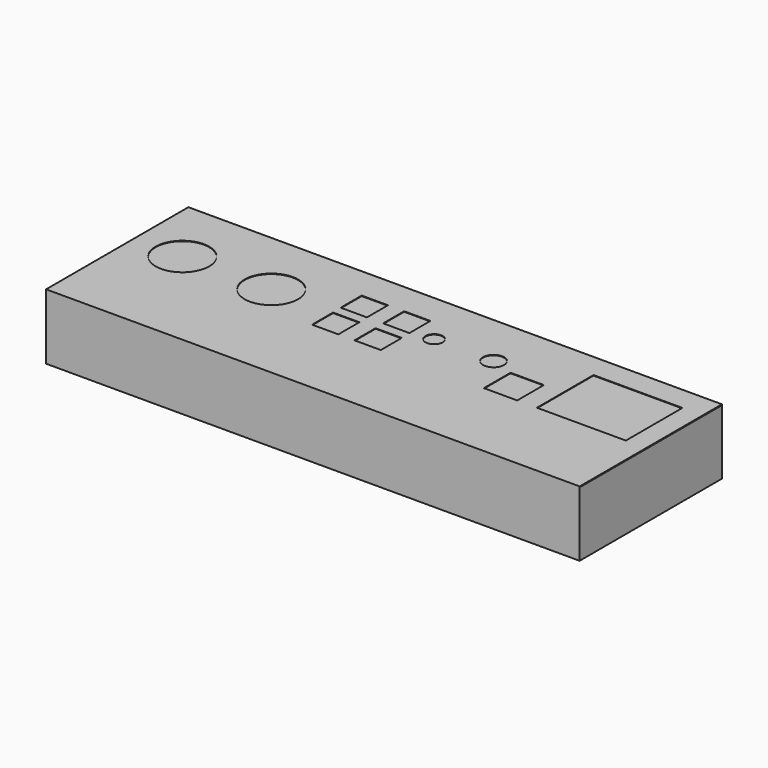
from build123d import *

# Parameters (mm, degrees)
F1_DEPTH = 209.55
F2_W     = 20.6375
F2_H     = 20.6375
F2_W_2   = 20.6374746
F2_W_3   = 69.85
F2_H_2   = 55.5625
F2_W_4   = 26.19375
F2_H_3   = 26.19375
F3_DEPTH = 0.4064


# Not quite as in the source:
# - the dataset's text gives a spline's control points without its knots; the knots are read off the source's solid


with BuildPart() as f1:
    # F0 (on Right) → F1 (new body, symmetric)
    with BuildSketch(Plane.YZ):
        Polygon((-139.7, 0), (0, 0), (0, 50.8), (-139.2936, 50.8), (-139.2936, 51.054), (0, 51.054), (0, 51.4604), (-139.7, 51.4604), align=None)
    extrude(amount=F1_DEPTH, both=True)

    # F2 (on face) → F3 (cut, through all)
    with BuildSketch(Plane.XY.offset(51.4604)):
        with Locations((-42.494652462, -64.131877524)):
            Rectangle(F2_W, F2_H)
        with Locations((-42.891171862, -35.556877524)):
            Rectangle(F2_W, F2_H)
        with Locations((-9.157152462, -64.131877524)):
            Rectangle(F2_W, F2_H)
        with Locations((-9.553684562, -35.556877524)):
            Rectangle(F2_W_2, F2_H)
        with Locations((158.720972538, -46.669377524)):
            Rectangle(F2_W_3, F2_H_2)
        with Locations((95.220972538, -61.353752524)):
            Rectangle(F2_W_4, F2_H_3)
        with BuildLine():
            add(Edge.make_bspline(
                [(22.455052538, -37.929872524), (21.206185338, -36.680675124), (19.450918338, -35.953752524), (17.684246738, -35.953752524)],
                knots=[7, 7, 7, 7, 8, 8, 8, 8], degree=3))
            add(Edge.make_bspline(
                [(17.684246738, -35.953752524), (15.918311738, -35.953752524), (14.163044738, -36.680675124), (12.913847338, -37.929872524)],
                knots=[0, 0, 0, 0, 1, 1, 1, 1], degree=3))
            add(Edge.make_bspline(
                [(12.913847338, -37.929872524), (11.664980138, -39.178384124), (10.937371738, -40.933981324), (10.937371738, -42.700627524), (10.937371738, -44.466587924), (11.664980138, -46.222235924), (12.913847338, -47.471407924)],
                knots=[1, 1, 1, 1, 2, 2, 2, 3, 3, 3, 3], degree=3))
            add(Edge.make_bspline(
                [(12.913847338, -47.471407924), (14.163044738, -48.719894124), (15.918311738, -49.447502524), (17.684246738, -49.447502524), (19.450918338, -49.447502524), (21.206185338, -48.719894124), (22.455052538, -47.471407924)],
                knots=[3, 3, 3, 3, 4, 4, 4, 5, 5, 5, 5], degree=3))
            add(Edge.make_bspline(
                [(22.455052538, -47.471407924), (23.704224538, -46.222235924), (24.431121738, -44.466587924), (24.431121738, -42.700627524), (24.431121738, -40.933981324), (23.704224538, -39.178384124), (22.455052538, -37.929872524)],
                knots=[5, 5, 5, 5, 6, 6, 6, 7, 7, 7, 7], degree=3))
        make_face()
        with BuildLine():
            add(Edge.make_bspline(
                [(-86.755549462, -38.542393524), (-90.649191662, -34.648751324), (-96.122028062, -32.381877524), (-101.629027462, -32.381877524)],
                knots=[7, 7, 7, 7, 8, 8, 8, 8], degree=3))
            add(Edge.make_bspline(
                [(-101.629027462, -32.381877524), (-107.135341062, -32.381877524), (-112.608533062, -34.648751324), (-116.502175262, -38.542393524)],
                knots=[0, 0, 0, 0, 1, 1, 1, 1], degree=3))
            add(Edge.make_bspline(
                [(-116.502175262, -38.542393524), (-120.395868262, -42.436035724), (-122.663402462, -47.908922924), (-122.663402462, -53.416252524), (-122.663402462, -58.922896324), (-120.395868262, -64.395783524), (-116.502175262, -68.290136924)],
                knots=[1, 1, 1, 1, 2, 2, 2, 3, 3, 3, 3], degree=3))
            add(Edge.make_bspline(
                [(-116.502175262, -68.290136924), (-112.608533062, -72.183779124), (-107.135341062, -74.450627524), (-101.629027462, -74.450627524), (-96.122028062, -74.450627524), (-90.649191662, -72.183779124), (-86.755549462, -68.290136924)],
                knots=[3, 3, 3, 3, 4, 4, 4, 5, 5, 5, 5], degree=3))
            add(Edge.make_bspline(
                [(-86.755549462, -68.290136924), (-82.861551662, -64.395783524), (-80.594652462, -58.922896324), (-80.594652462, -53.416252524), (-80.594652462, -47.908922924), (-82.861551662, -42.436035724), (-86.755549462, -38.542393524)],
                knots=[5, 5, 5, 5, 6, 6, 6, 7, 7, 7, 7], degree=3))
        make_face()
        with BuildLine():
            add(Edge.make_bspline(
                [(-156.605549462, -38.542393524), (-160.499191662, -34.648751324), (-165.972028062, -32.381877524), (-171.479027462, -32.381877524)],
                knots=[7, 7, 7, 7, 8, 8, 8, 8], degree=3))
            add(Edge.make_bspline(
                [(-171.479027462, -32.381877524), (-176.985341062, -32.381877524), (-182.458355262, -34.648751324), (-186.352353062, -38.542393524), (-190.246350862, -42.436035724), (-192.513402462, -47.908922924), (-192.513402462, -53.416252524), (-192.513402462, -58.922896324), (-190.246350862, -64.395783524), (-186.352353062, -68.290136924)],
                knots=[0, 0, 0, 0, 1, 1, 1, 2, 2, 2, 3, 3, 3, 3], degree=3))
            add(Edge.make_bspline(
                [(-186.352353062, -68.290136924), (-182.458355262, -72.183779124), (-176.985341062, -74.450627524), (-171.479027462, -74.450627524), (-165.972028062, -74.450627524), (-160.499191662, -72.183779124), (-156.605549462, -68.290136924)],
                knots=[3, 3, 3, 3, 4, 4, 4, 5, 5, 5, 5], degree=3))
            add(Edge.make_bspline(
                [(-156.605549462, -68.290136924), (-152.711551662, -64.395783524), (-150.444652462, -58.922896324), (-150.444652462, -53.416252524), (-150.444652462, -47.908922924), (-152.711551662, -42.436035724), (-156.605549462, -38.542393524)],
                knots=[5, 5, 5, 5, 6, 6, 6, 7, 7, 7, 7], degree=3))
        make_face()
        with BuildLine():
            add(Edge.make_bspline(
                [(70.202658338, -36.807471924), (68.659963938, -35.264066324), (66.491972338, -34.366252524), (64.309502738, -34.366252524)],
                knots=[7, 7, 7, 7, 8, 8, 8, 8], degree=3))
            add(Edge.make_bspline(
                [(64.309502738, -34.366252524), (62.127363338, -34.366252524), (59.959016138, -35.264066324), (58.416321738, -36.807471924)],
                knots=[0, 0, 0, 0, 1, 1, 1, 1], degree=3))
            add(Edge.make_bspline(
                [(58.416321738, -36.807471924), (56.873271738, -38.350166324), (55.975127738, -40.518513524), (55.975127738, -42.700627524), (55.975127738, -44.882766924), (56.873271738, -47.051114124), (58.416321738, -48.593808524)],
                knots=[1, 1, 1, 1, 2, 2, 2, 3, 3, 3, 3], degree=3))
            add(Edge.make_bspline(
                [(58.416321738, -48.593808524), (59.959016138, -50.136553724), (62.127363338, -51.035002524), (64.309502738, -51.035002524), (66.491972338, -51.035002524), (68.659963938, -50.136553724), (70.202658338, -48.593808524)],
                knots=[3, 3, 3, 3, 4, 4, 4, 5, 5, 5, 5], degree=3))
            add(Edge.make_bspline(
                [(70.202658338, -48.593808524), (71.745759138, -47.051114124), (72.643877738, -44.882766924), (72.643877738, -42.700627524), (72.643877738, -40.518513524), (71.745759138, -38.350166324), (70.202658338, -36.807471924)],
                knots=[5, 5, 5, 5, 6, 6, 6, 7, 7, 7, 7], degree=3))
        make_face()
    extrude(amount=-F3_DEPTH, mode=Mode.SUBTRACT)


solid = f1.part
